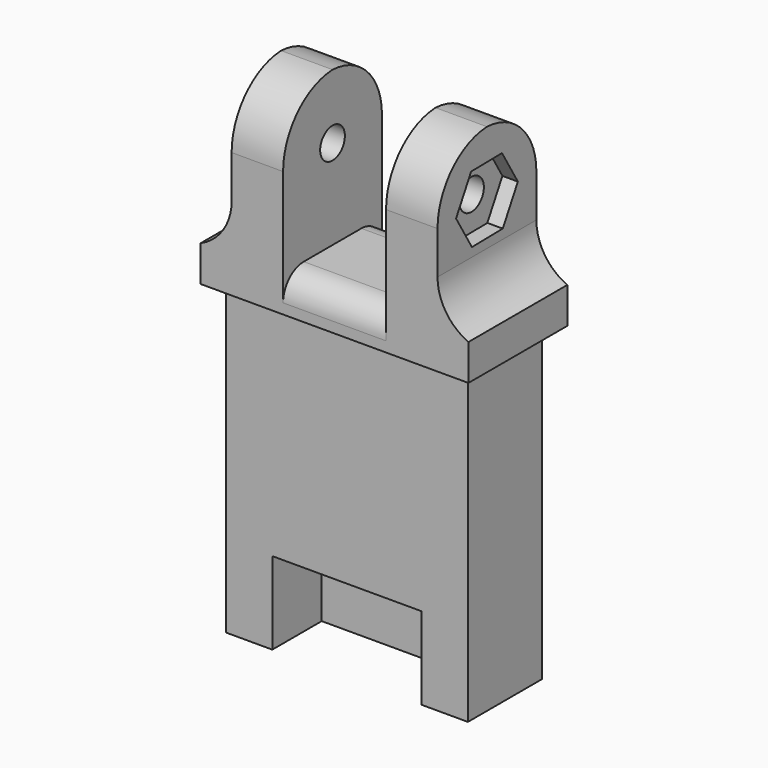
from build123d import *

# Parameters (mm, degrees)
F0_W         = 23.5
F0_H         = 9
F2_DEPTH     = 30
F3_W         = 26
F3_H         = 12
F3_W_2       = 23.5
F3_H_2       = 9
F4_DEPTH     = 3.5
F5_W         = 5
F5_H         = 12
F7_DEPTH     = 15
F8_T1_DEPTH  = 36.3847763109
F8_T3_DEPTH  = 36.3847763109
F12_DEPTH    = 1.5
F9_R         = 1.5
F14_DEPTH    = 25
F15_W        = 7.25
F15_H        = 8
F17_DEPTH    = 6
F18_T1_DEPTH = 12
F19_R        = 2.5
F9_R_2       = 2.75
F20_DEPTH    = 2


# Not quite as in the source:
# - a fillet or chamfer that OpenCascade refuses, or shapes differently, is made with other operations: its cross-section is extruded or revolved along the edge and cut away or added


with BuildPart() as f2:
    # F0 (on Top) → F2 (new body)
    with BuildSketch(Plane.XY):
        Rectangle(F0_W, F0_H)
    extrude(amount=-F2_DEPTH)

    # F15 (on face) → F17 (cut)
    with BuildSketch(Plane.XZ.offset(4.5)):
        with Locations((3.625, -26)):
            Rectangle(F15_W, F15_H)
        with Locations((-3.625, -26)):
            Rectangle(F15_W, F15_H)
    extrude(amount=-F17_DEPTH, mode=Mode.SUBTRACT)


with BuildPart() as f4:
    # F3 (on face) → F4 (new body)
    with BuildSketch(Plane.XY):
        Rectangle(F3_W, F3_H)
        Rectangle(F3_W_2, F3_H_2, mode=Mode.SUBTRACT)
        Rectangle(F3_W_2, F3_H_2)
    extrude(amount=F4_DEPTH)

    # F5 (on face) → F7 (join)
    with BuildSketch(Plane.XY.offset(3.5)):
        with Locations((-7.5, 0)):
            Rectangle(F5_W, F5_H)
        with Locations((7.5, 0)):
            Rectangle(F5_W, F5_H)
    extrude(amount=F7_DEPTH)

    # F8: fillet of radius 6.2769552622 on 4 edges, made by hand

    # F8_s2 → F8_t1 (cut)
    with BuildSketch(Plane.YZ.offset(-25.6923881554)):
        with BuildLine():
            ThreePointArc((-6, 12.2230447378), (-4.1615223689, 16.6615223689), (0.2769552622, 18.5))
            Line((0.2769552622, 18.5), (-6, 18.5))
            Line((-6, 18.5), (-6, 12.2230447378))
        make_face()
        with BuildLine():
            ThreePointArc((6, 12.2230447378), (4.1615223689, 16.6615223689), (-0.2769552622, 18.5))
            Line((-0.2769552622, 18.5), (6, 18.5))
            Line((6, 18.5), (6, 12.2230447378))
        make_face()
    extrude(amount=F8_T1_DEPTH, mode=Mode.SUBTRACT)

    # F8_s4 → F8_t3 (cut)
    with BuildSketch(Plane.YZ.offset(-10.6923881554)):
        with BuildLine():
            ThreePointArc((6, 12.2230447378), (4.1615223689, 16.6615223689), (-0.2769552622, 18.5))
            Line((-0.2769552622, 18.5), (6, 18.5))
            Line((6, 18.5), (6, 12.2230447378))
        make_face()
        with BuildLine():
            ThreePointArc((-6, 12.2230447378), (-4.1615223689, 16.6615223689), (0.2769552622, 18.5))
            Line((0.2769552622, 18.5), (-6, 18.5))
            Line((-6, 18.5), (-6, 12.2230447378))
        make_face()
    extrude(amount=F8_T3_DEPTH, mode=Mode.SUBTRACT)

    # F10 (on face) → F12 (cut)
    with BuildSketch(Plane.YZ.offset(10)):
        Polygon((1.922952101, 9.0003768135), (3.7523883409, 12.2770361454), (1.8294362399, 15.4997040697), (-1.922952101, 15.4457126622), (-3.7523883409, 12.1690533302), (-1.8294362399, 8.9463854059), align=None)
    extrude(amount=-F12_DEPTH, mode=Mode.SUBTRACT)

    # F9 (on face) → F14 (cut)
    with BuildSketch(Plane(origin=(-10, 0, 0), x_dir=(0, -1, 0), z_dir=(-1, 0, 0))):
        with Locations((0, 12.2230447378)):
            Circle(F9_R)
    extrude(amount=-F14_DEPTH, mode=Mode.SUBTRACT)

    # F18: fillet of radius 5 on 2 edges, made by hand

    # F18_s2 → F18_t1 (join)
    with BuildSketch(Plane.XZ.offset(-6)):
        with BuildLine():
            ThreePointArc((13, 3.5), (10.8166998673, 5.3439629074), (10, 8.082575695))
            Line((10, 8.082575695), (10, 3.5))
            Line((10, 3.5), (13, 3.5))
        make_face()
        with BuildLine():
            ThreePointArc((-10, 8.082575695), (-10.8166998673, 5.3439629074), (-13, 3.5))
            Line((-13, 3.5), (-10, 3.5))
            Line((-10, 3.5), (-10, 8.082575695))
        make_face()
    extrude(amount=F18_T1_DEPTH)

    # F19
    f19_edges = [f4.edges().sort_by_distance(p)[0] for p in [
        (0, 6, 3.5),
        (0, -6, 3.5),
    ]]
    fillet(f19_edges, radius=F19_R)

    # F9 (on face) → F20 (cut)
    with BuildSketch(Plane(origin=(-10, 0, 0), x_dir=(0, -1, 0), z_dir=(-1, 0, 0))):
        with Locations((0, 12.2230447378)):
            Circle(F9_R_2)
        with Locations((0, 12.2230447378)):
            Circle(F9_R, mode=Mode.SUBTRACT)
    extrude(amount=-F20_DEPTH, mode=Mode.SUBTRACT)


solid = Compound([f2.part, f4.part])
